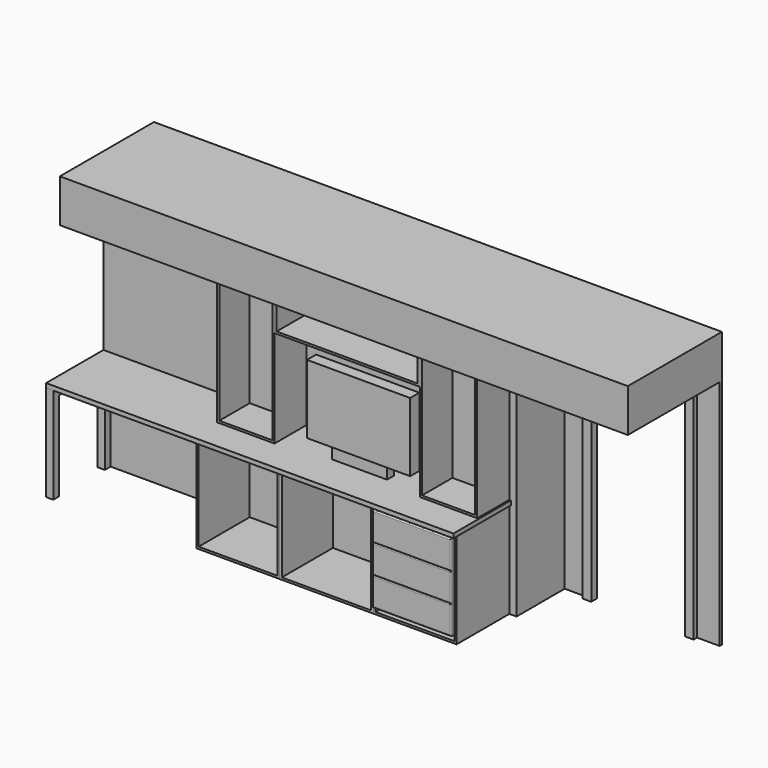
from build123d import *

# Parameters (mm, degrees)
F0_W      = 5029.2
F0_H      = 2438.4
F1_DEPTH  = 25.4
F2_W      = 3657.6
F2_H      = 2057.4
F3_DEPTH  = 533.4
F5_DEPTH  = 1016
F6_W      = 830.1289733465
F6_H      = 1981.2
F7_DEPTH  = 25.4
F9_DEPTH  = 38.1
F10_W     = 3606.8
F10_H     = 38.1
F11_DEPTH = 635
F12_W     = 63.5
F12_H     = 850.9
F13_DEPTH = 63.5
F14_W     = 508
F14_H     = 63.5
F15_DEPTH = 63.5
F17_DEPTH = 63.5
F18_W     = 736.6
F18_H     = 850.9
F19_DEPTH = 584.2
F20_T     = -19.05
F21_W     = 829.7205785751
F21_H     = 850.9
F22_DEPTH = 584.2
F23_T     = -19.05
F24_W     = 736.6
F24_H     = 850.9
F25_DEPTH = 584.2
F26_T     = -19.05
F27_W     = 698.5
F27_H     = 254
F28_DEPTH = 38.1
F29_W     = 485.3785143141
F29_H     = 76.2
F30_DEPTH = 101.6
F31_W     = 914.4
F31_H     = 101.6
F32_DEPTH = 609.6
F33_W     = 508
F33_H     = 1167.0816213608
F34_DEPTH = 355.6
F35_T     = -19.05
F36_W     = 508
F36_H     = 1168.4
F37_DEPTH = 355.6
F38_T     = -19.05
F39_W     = 1286.9205785751
F39_H     = 307.5614840508
F40_DEPTH = 355.6
F41_T     = -19.05
F42_R     = 10.16
F43_W     = 698.5
F43_H     = 254
F44_DEPTH = 38.1
F45_R     = 10.15999
F46_W     = 698.5
F46_H     = 254
F47_DEPTH = 38.1
F48_R     = 10.1599


# Not quite as in the source:
# - a fillet or chamfer is up to 0.001 mm smaller than in the source, because OpenCascade refuses the exact size


with BuildPart() as f1:
    # F0 (on Front) → F1 (new body)
    with BuildSketch(Plane.XZ):
        Rectangle(F0_W, F0_H)
    extrude(amount=-F1_DEPTH)

    # F2 (on face) → F3 (join)
    with BuildSketch(Plane.XZ):
        with Locations((-685.8, -190.5)):
            Rectangle(F2_W, F2_H)
    extrude(amount=F3_DEPTH)

    # F4 (on face) → F5 (join)
    with BuildSketch(Plane.XZ):
        Polygon((-2514.6, 1219.2), (-2514.6, 838.2), (1143, 838.2), (2514.6, 838.2), (2514.6, 1219.2), align=None)
    extrude(amount=F5_DEPTH)

    # F6 (on face) → F7 (cut)
    with BuildSketch(Plane.XZ):
        with Locations((1823.4765855578, -228.6)):
            Rectangle(F6_W, F6_H)
    extrude(amount=-F7_DEPTH, mode=Mode.SUBTRACT)

    # F8 (on face) → F9 (join)
    with BuildSketch(Plane.XZ):
        Polygon((2314.7410722311, 838.2), (1332.2120988846, 838.2), (1332.2120988846, -1219.2), (1408.4120988846, -1219.2), (1408.4120988846, 762), (2238.5410722311, 762), (2238.5410722311, -1219.2), (2314.7410722311, -1219.2), align=None)
    extrude(amount=F9_DEPTH)


with BuildPart() as f11:
    # F10 (on face) → F11 (new body)
    with BuildSketch(Plane.XZ.offset(533.4)):
        with Locations((-711.2, -349.25)):
            Rectangle(F10_W, F10_H)
    extrude(amount=F11_DEPTH)

    # F29 (on face) → F30 (join)
    with BuildSketch(Plane.XY.offset(-330.2)):
        with Locations((-12.7, -787.4)):
            Rectangle(F29_W, F29_H)
    extrude(amount=F30_DEPTH)

    # F31 (on face) → F32 (join)
    with BuildSketch(Plane.XY.offset(-228.6)):
        with Locations((-12.7, -786.4327430725)):
            Rectangle(F31_W, F31_H)
    extrude(amount=F32_DEPTH)


with BuildPart() as f13:
    # F12 (on face) → F13 (new body)
    with BuildSketch(Plane.XZ.offset(533.4)):
        with Locations((-2482.85, -793.75)):
            Rectangle(F12_W, F12_H)
    extrude(amount=F13_DEPTH)


with BuildPart() as f15:
    # F14 (on face) → F15 (new body)
    with BuildSketch(Plane(origin=(-2514.6, 0, 0), x_dir=(0, -1, 0), z_dir=(-1, 0, 0))):
        with Locations((850.9, -400.05)):
            Rectangle(F14_W, F14_H)
    extrude(amount=-F15_DEPTH)


with BuildPart() as f17:
    # F16 (on face) → F17 (new body)
    with BuildSketch(Plane(origin=(-2514.6, 0, 0), x_dir=(0, -1, 0), z_dir=(-1, 0, 0))):
        Polygon((1168.4, -368.3), (1104.9, -368.3), (1104.9, -431.8), (1104.9, -1219.2), (1168.4, -1219.2), align=None)
    extrude(amount=-F17_DEPTH)


with BuildPart() as f19:
    # F18 (on face) → F19 (new body)
    with BuildSketch(Plane.XZ.offset(533.4)):
        with Locations((711.2, -793.75)):
            Rectangle(F18_W, F18_H)
    extrude(amount=F19_DEPTH)

    # F20
    f20_openings = [f19.faces().sort_by_distance(p)[0] for p in [
        (711.2, -1117.6, -793.75),
    ]]
    offset(amount=F20_T, openings=f20_openings)



with BuildPart() as f22:
    # F21 (on face) → F22 (new body)
    with BuildSketch(Plane.XZ.offset(533.4)):
        with Locations((-71.9602892876, -793.75)):
            Rectangle(F21_W, F21_H)
    extrude(amount=F22_DEPTH)

    # F23
    f23_openings = [f22.faces().sort_by_distance(p)[0] for p in [
        (-71.960289, -1117.6, -793.75),
    ]]
    offset(amount=F23_T, openings=f23_openings)


with BuildPart() as f25:
    # F24 (on face) → F25 (new body)
    with BuildSketch(Plane.XZ.offset(533.4)):
        with Locations((-855.1205785751, -793.75)):
            Rectangle(F24_W, F24_H)
    extrude(amount=F25_DEPTH)

    # F26
    f26_openings = [f25.faces().sort_by_distance(p)[0] for p in [
        (-855.120579, -1117.6, -793.75),
    ]]
    offset(amount=F26_T, openings=f26_openings)


with BuildPart() as f28:
    # F27 (on face) → F28 (new body)
    with BuildSketch(Plane.XZ.offset(1117.6)):
        with Locations((711.2, -514.35)):
            Rectangle(F27_W, F27_H)
    extrude(amount=F28_DEPTH)

    # F42
    f42_edges = [f28.edges().sort_by_distance(p)[0] for p in [
        (711.2, -1155.7, -387.35),
        (361.95, -1155.7, -514.35),
        (711.2, -1155.7, -641.35),
        (1060.45, -1155.7, -514.35),
    ]]
    fillet(f42_edges, radius=F42_R)


with BuildPart() as f34:
    # F33 (on face) → F34 (new body)
    with BuildSketch(Plane.XZ.offset(533.4)):
        with Locations((825.5, 254.6591893196)):
            Rectangle(F33_W, F33_H)
    extrude(amount=F34_DEPTH)

    # F35
    f35_openings = [f34.faces().sort_by_distance(p)[0] for p in [
        (825.5, -889, 254.659189),
    ]]
    offset(amount=F35_T, openings=f35_openings)


with BuildPart() as f37:
    # F36 (on face) → F37 (new body)
    with BuildSketch(Plane.XZ.offset(533.4)):
        with Locations((-969.4205785751, 254)):
            Rectangle(F36_W, F36_H)
    extrude(amount=F37_DEPTH)

    # F38
    f38_openings = [f37.faces().sort_by_distance(p)[0] for p in [
        (-969.420579, -889, 254),
    ]]
    offset(amount=F38_T, openings=f38_openings)


with BuildPart() as f40:
    # F39 (on face) → F40 (new body)
    with BuildSketch(Plane.XZ.offset(533.4)):
        with Locations((-71.9602892876, 684.4192579746)):
            Rectangle(F39_W, F39_H)
    extrude(amount=F40_DEPTH)

    # F41
    f41_openings = [f40.faces().sort_by_distance(p)[0] for p in [
        (-71.960289, -889, 684.419258),
    ]]
    offset(amount=F41_T, openings=f41_openings)


with BuildPart() as f19_1:
    add(f19.part)

    add(f28.part)  # F44 merges F28
    # F43 (on face) → F44 (join)
    with BuildSketch(Plane.XZ.offset(1117.6)):
        with Locations((711.2, -768.35)):
            Rectangle(F43_W, F43_H)
    extrude(amount=F44_DEPTH)

    # F45 (radius 10.16 in the source; OpenCascade refuses exactly that, so slightly less here)
    f45_edges = [f19_1.edges().sort_by_distance(p)[0] for p in [
        (1060.45, -1155.7, -768.35),
        (711.2, -1155.7, -641.35),
        (361.95, -1155.7, -768.35),
        (711.2, -1155.7, -895.35),
    ]]
    fillet(f45_edges, radius=F45_R)

    # F46 (on face) → F47 (join)
    with BuildSketch(Plane.XZ.offset(1117.6)):
        with Locations((711.2, -1022.35)):
            Rectangle(F46_W, F46_H)
    extrude(amount=F47_DEPTH)

    # F48 (radius 10.16 in the source; OpenCascade refuses exactly that, so slightly less here)
    f48_edges = [f19_1.edges().sort_by_distance(p)[0] for p in [
        (711.2, -1155.7, -895.35),
        (361.95, -1155.7, -1022.35),
        (711.2, -1155.7, -1149.35),
        (1060.45, -1155.7, -1022.35),
    ]]
    fillet(f48_edges, radius=F48_R)


solid = Compound([f1.part, f11.part, f13.part, f15.part, f17.part, f22.part, f25.part, f34.part, f37.part, f40.part, f19_1.part])
